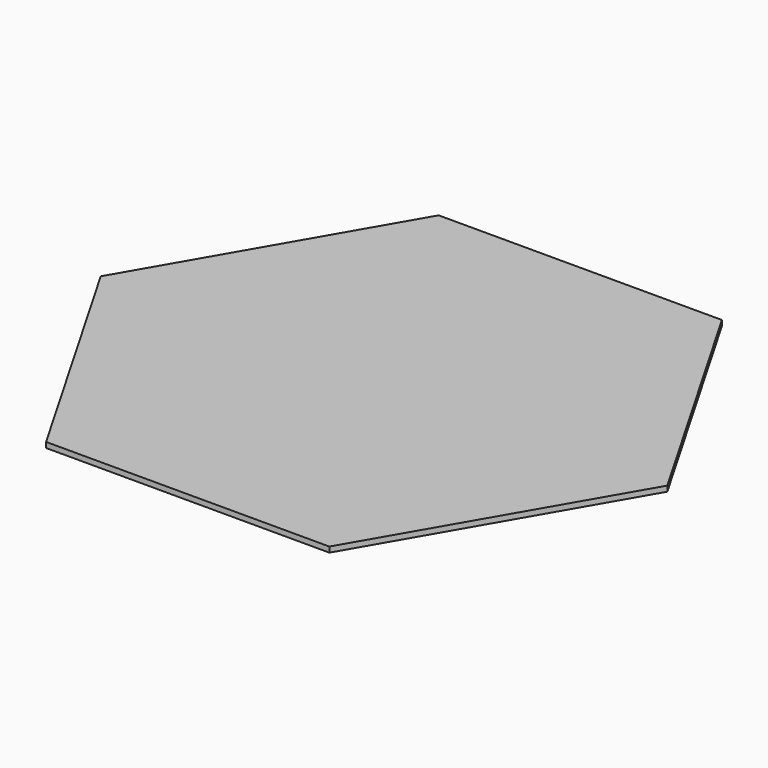
from build123d import *

# Parameters (mm, degrees)
F2_DEPTH = 5.08


# Not quite as in the source:
# - the program builds the solid bodies; features that only make, move or delete a surface that nothing else refers to are left out


with BuildPart() as f2:
    # F0 (on Top) → F2 (new body)
    with BuildSketch(Plane.XY):
        Polygon((266.7, 0), (133.35, 230.9689751893), (-133.35, 230.9689751893), (-266.7, 0), (-133.35, -230.9689751893), (133.35, -230.9689751893), align=None)
    extrude(amount=F2_DEPTH)


solid = f2.part
